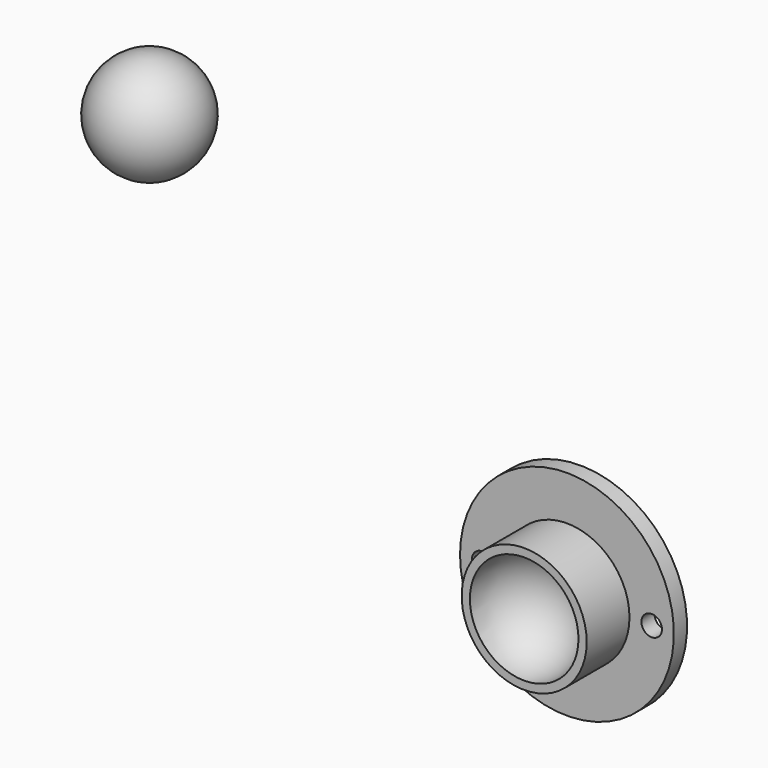
from build123d import *

# Parameters (mm, degrees)
F1_DEPTH = 4.1275
F0_R     = 8.382
F2_DEPTH = 12.3825
F3_DEPTH = 1.5875


# Not quite as in the source:
# - a length typed as a fraction of an inch, garbled in the dataset ("3 / 203.2 mm" for 3/8 in), is restored


with BuildPart() as f1:
    # F0 (on Front) → F1 (new body)
    with BuildSketch(Plane.XZ):
        with BuildLine():
            ThreePointArc((-9.652, 0), (0, 9.652), (9.652, 0))
            Line((9.652, 0), (11.4935, 0))
            ThreePointArc((11.4935, 0), (13.081, 1.5875), (14.6685, 0))
            Line((14.6685, 0), (16.51, 0))
            ThreePointArc((16.51, 0), (0, 16.51), (-16.51, 0))
            Line((-16.51, 0), (-14.6685, 0))
            ThreePointArc((-14.6685, 0), (-13.081, 1.5875), (-11.4935, 0))
            Line((-11.4935, 0), (-9.652, 0))
        make_face()
        with BuildLine():
            Line((11.4935, 0), (9.652, 0))
            ThreePointArc((9.652, 0), (0, -9.652), (-9.652, 0))
            Line((-9.652, 0), (-11.4935, 0))
            ThreePointArc((-11.4935, 0), (-13.081, -1.5875), (-14.6685, 0))
            Line((-14.6685, 0), (-16.51, 0))
            ThreePointArc((-16.51, 0), (0, -16.51), (16.51, 0))
            Line((16.51, 0), (14.6685, 0))
            ThreePointArc((14.6685, 0), (13.081, -1.5875), (11.4935, 0))
        make_face()
    extrude(amount=F1_DEPTH)

    # F0 (on Front) → F2 (join)
    with BuildSketch(Plane.XZ):
        with BuildLine():
            ThreePointArc((-9.652, 0), (0, -9.652), (9.652, 0))
            ThreePointArc((9.652, 0), (0, 9.652), (-9.652, 0))
        make_face()
        Circle(F0_R, mode=Mode.SUBTRACT)
        Circle(F0_R)
    extrude(amount=F2_DEPTH)

    # F0 (on Front) → F3 (cut)
    with BuildSketch(Plane.XZ):
        with BuildLine():
            ThreePointArc((-9.652, 0), (0, -9.652), (9.652, 0))
            ThreePointArc((9.652, 0), (0, 9.652), (-9.652, 0))
        make_face()
        Circle(F0_R, mode=Mode.SUBTRACT)
        Circle(F0_R)
        with BuildLine():
            ThreePointArc((-9.652, 0), (0, 9.652), (9.652, 0))
            Line((9.652, 0), (11.4935, 0))
            ThreePointArc((11.4935, 0), (13.081, 1.5875), (14.6685, 0))
            Line((14.6685, 0), (16.51, 0))
            ThreePointArc((16.51, 0), (0, 16.51), (-16.51, 0))
            Line((-16.51, 0), (-14.6685, 0))
            ThreePointArc((-14.6685, 0), (-13.081, 1.5875), (-11.4935, 0))
            Line((-11.4935, 0), (-9.652, 0))
        make_face()
        with BuildLine():
            Line((11.4935, 0), (9.652, 0))
            ThreePointArc((9.652, 0), (0, -9.652), (-9.652, 0))
            Line((-9.652, 0), (-11.4935, 0))
            ThreePointArc((-11.4935, 0), (-13.081, -1.5875), (-14.6685, 0))
            Line((-14.6685, 0), (-16.51, 0))
            ThreePointArc((-16.51, 0), (0, -16.51), (16.51, 0))
            Line((16.51, 0), (14.6685, 0))
            ThreePointArc((14.6685, 0), (13.081, -1.5875), (11.4935, 0))
        make_face()
    extrude(amount=F3_DEPTH, mode=Mode.SUBTRACT)

    # F4 (on face) → F5 (revolve, cut)
    with BuildSketch(Plane.XZ.offset(12.3825)):
        with BuildLine():
            Line((0, -8.382), (0, 8.382))
            ThreePointArc((0, 8.382), (-8.382, 0), (0, -8.382))
        make_face()
    revolve(axis=Axis((0, -12.3825, 0), (0, 0, -1)), mode=Mode.SUBTRACT)


with BuildPart() as f7:
    # F6 (on Front) → F7 (revolve)
    with BuildSketch(Plane.XZ):
        with BuildLine():
            Line((-67.7581787605, 33.248559798), (-67.7581787605, 49.758559798))
            ThreePointArc((-67.7581787605, 49.758559798), (-76.0131787605, 41.503559798), (-67.7581787605, 33.248559798))
        make_face()
    revolve(axis=Axis((-67.7581787605, 0, 41.503559798), (0, 0, -1)))


solid = Compound([f1.part, f7.part])
